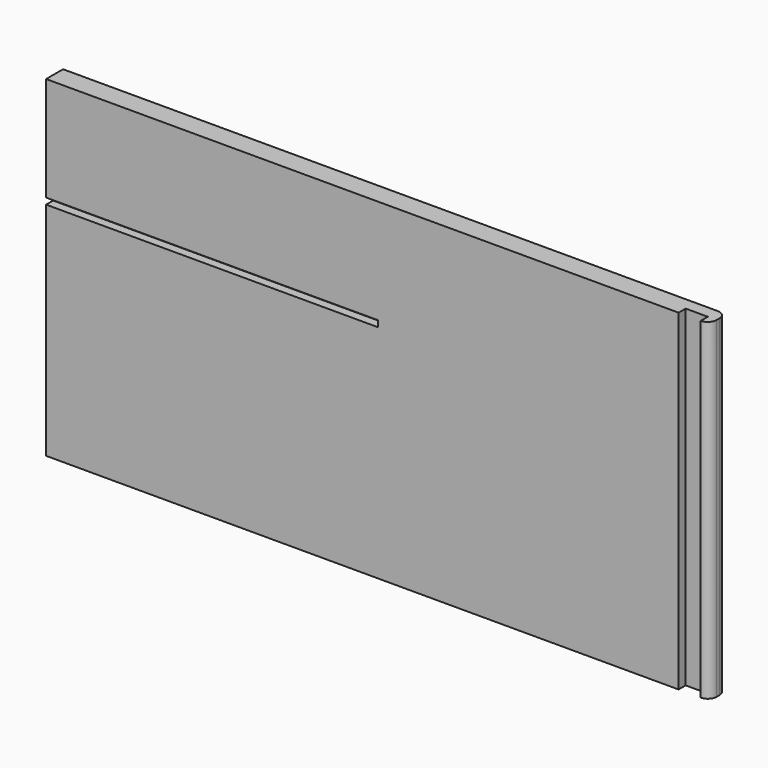
from build123d import *

# Parameters (mm, degrees)
F0_W     = 150
F0_H     = 75
F1_DEPTH = 4.8
F2_W     = 5
F2_H     = 75
F2_W_2   = 75
F2_H_2   = 1.4
F3_DEPTH = 2
F4_R     = 1.99999


# Not quite as in the source:
# - a fillet or chamfer is up to 0.001 mm smaller than in the source, because OpenCascade refuses the exact size


with BuildPart() as f1:
    # F0 (on Front) → F1 (new body)
    with BuildSketch(Plane.XZ):
        Rectangle(F0_W, F0_H)
    extrude(amount=F1_DEPTH)

    # F2 (on face) → F3 (cut)
    with BuildSketch(Plane.XZ.offset(4.8)):
        with Locations((70.5, 0)):
            Rectangle(F2_W, F2_H)
        with Locations((-37.5, 13.2)):
            Rectangle(F2_W_2, F2_H_2)
    extrude(amount=-F3_DEPTH, mode=Mode.SUBTRACT)

    # F4 (radius 2 in the source; OpenCascade refuses exactly that, so slightly less here)
    f4_edges = [f1.edges().sort_by_distance(p)[0] for p in [
        (75, 0, 0),
        (75, -4.8, 0),
    ]]
    fillet(f4_edges, radius=F4_R)


solid = f1.part
